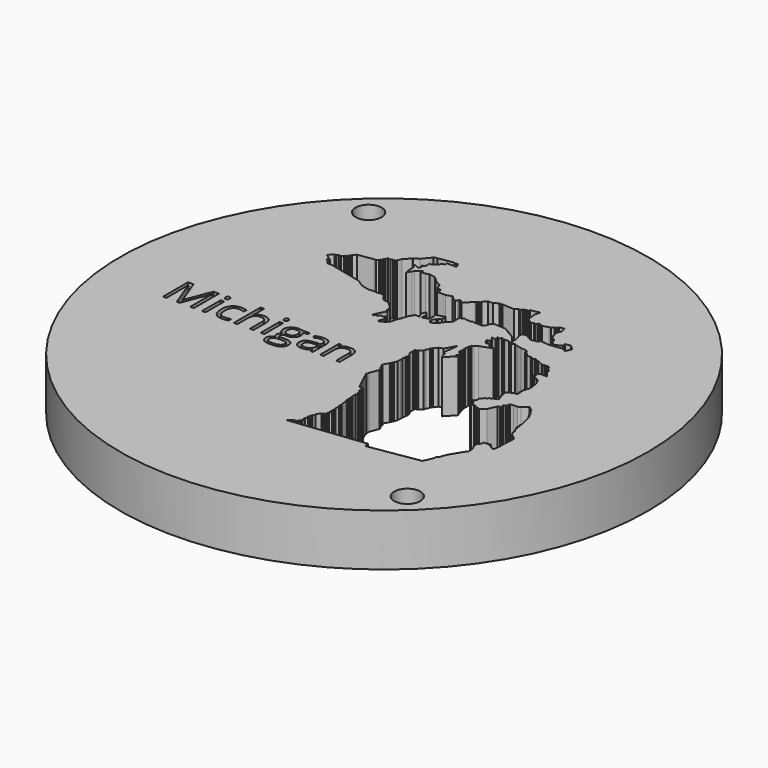
from build123d import *

# Parameters (mm, degrees)
F0_R         = 25.4
F0_R_2       = 1.25
F1_DEPTH     = 5
F2_TEXT_SIZE = 4.2111256337
F3_DEPTH     = 25


# Not quite as in the source:
# - Text() gives the source's letters only with a copy of the font that has no kerning and outlines rounded to 1/6400 em; it was checked with that copy


with BuildPart() as f1:
    # F0 (on Top) → F1 (new body)
    with BuildSketch(Plane.XY):
        Circle(F0_R)
        with Locations((15.783349916, -16.9354174861)):
            Circle(F0_R_2, mode=Mode.SUBTRACT)
        with Locations((-15.3492664, 17.3298159535)):
            Circle(F0_R_2, mode=Mode.SUBTRACT)
    extrude(amount=F1_DEPTH)

    # F2 (on face) → F3 (cut)
    with BuildSketch(Plane.XY.offset(5)):
        Polygon((-7.1277720854, 12.4056404456), (-7.3109893128, 12.8393787891), (-6.7987288348, 12.5963352621), (-6.6902944818, 12.9216387868), (-6.8395042811, 13.0705927815), (-6.5855989233, 13.1534645334), (-6.5736236811, 13.2494844339), (-6.5108160488, 13.3478995413), (-6.6192508675, 13.6918993667), (-6.3575119711, 13.6133776978), (-6.1593381688, 13.7953237279), (-5.796642974, 14.1817247495), (-5.5685560219, 14.3312895671), (-5.6059476919, 14.5182460546), (-5.0413394347, 14.5257245749), (-4.9815131351, 14.607985504), (-4.888035357, 14.5182460546), (-4.663687665, 14.5406806841), (-4.8581222072, 14.9893760681), (-4.9515999854, 14.7986812517), (-4.9927304499, 14.9519853294), (-5.0712525845, 14.8285934702), (-5.0824698992, 14.9220721796), (-5.2972559509, 14.9541556042), (-6.641685497, 14.735115692), (-6.7274633534, 14.6680477367), (-6.7821381753, 14.7193682406), (-6.9744680077, 14.6565940231), (-7.0342938416, 14.5444199443), (-7.6288152486, 13.826508075), (-8.0924667418, 13.5759860277), (-8.1448216866, 13.4778581533), (-8.6458576843, 12.9440743476), (-8.8066402823, 12.5514650717), (-8.9188143611, 12.4542480335), (-9.1095101088, 12.4617265537), (-9.2927273363, 12.3794656247), (-9.5656830817, 12.4093787745), (-9.6329879016, 12.2037269175), (-9.7414227203, 12.1027706191), (-9.7489003092, 11.9158150628), (-9.8573351279, 11.8709448725), (-9.8947267979, 11.7475539446), (-10.0913743195, 11.6190201435), (-10.2767857498, 11.6353798658), (-11.7455944419, 11.3960755989), (-12.0148109272, 11.1305983737), (-11.9587248191, 11.0072065145), (-12.0567845111, 11.0149033746), (-12.1308986992, 10.8987716958), (-12.0877359866, 10.7665282746), (-12.2728114948, 10.7828583568), (-12.3003042953, 10.6222052089), (-12.3801907504, 10.6257427085), (-12.5345503911, 10.4612940922), (-12.7769677552, 10.523354285), (-12.9007655011, 10.391465095), (-13.073738424, 10.3991246117), (-13.4813163299, 9.9649073364), (-13.1518466448, 9.7546427603), (-13.1106622391, 9.6284605448), (-12.9385474117, 9.6208390259), (-12.8557833095, 9.5680197237), (-13.0281141028, 9.384425357), (-13.0281141028, 9.3208597973), (-12.7850705758, 9.3283383176), (-12.7552073371, 9.1944148123), (-12.7252452075, 9.0105123818), (-12.628027238, 9.0591209009), (-12.5974396509, 8.9247867286), (-12.422375381, 8.9170346037), (-12.2466366738, 8.9394692332), (-9.0085528791, 8.1766871735), (-8.2644671202, 7.7018183656), (-7.505360331, 7.5182112386), (-7.1128155105, 7.5821662322), (-6.9782068022, 7.533557713), (-6.8809897639, 7.5859054923), (-6.7351637408, 7.4849487282), (-6.5631638281, 7.5933835469), (-5.8826426975, 7.4886879884), (-5.905077327, 7.2344271466), (-5.6844688952, 7.163383998), (-5.7442951947, 7.0512099192), (-5.6994254701, 6.9614709355), (-5.5909906514, 7.0175579749), (-5.5143811624, 6.8605176456), (-5.2619478665, 6.9016451016), (-5.127075726, 6.802898566), (-4.9927304499, 6.7969495431), (-4.2811993246, 6.0895033047), (-4.3982090428, 6.0379067436), (-4.3771734405, 5.9902025972), (-4.1589052416, 5.8808634058), (-4.3498775797, 5.7425163686), (-4.3245454219, 5.6649028218), (-4.1775836656, 5.658395121), (-4.6823825687, 4.6506910585), (-4.7160349786, 4.4824304059), (-4.6001221053, 4.4786911458), (-4.4909280854, 4.6080096089), (-4.3570785783, 4.6020825393), (-4.2486442253, 4.6510417404), (-4.1551659815, 4.8376475461), (-3.9420356043, 4.7441693023), (-3.7438618019, 4.8825168051), (-3.6466452293, 4.8899953254), (-3.5859393744, 4.7605300768), (-3.6802967079, 4.5721693896), (-3.6167316139, 4.4973869808), (-3.4922887951, 4.4772454448), (-3.7401227746, 4.2132129893), (-3.7401227746, 3.9963438176), (-3.6466452293, 3.9365179837), (-3.1156884506, 4.2917346582), (-3.0782972462, 4.4375606813), (-3.0118077362, 4.3613059405), (-2.9698626604, 4.4450387359), (-2.913775621, 4.6768649481), (-2.8142493157, 5.0720415796), (-2.6063358623, 5.4870885028), (-2.6290135387, 5.6262802047), (-2.5199085008, 5.7425163686), (-2.5199085008, 5.9331770969), (-2.4163748255, 6.0434777529), (-2.2987988717, 6.2781885764), (-2.206857817, 6.4617257707), (-2.0555970742, 6.4550277039), (-1.9404778719, 6.4926012709), (-1.8345903468, 6.4395580129), (-1.7658638535, 6.5127764829), (-1.9040555406, 6.7148180333), (-1.9479481664, 6.849297788), (-1.9479481664, 6.9602626832), (-1.9405520285, 7.1272877898), (-1.8653408393, 7.1239573185), (-1.8818918278, 7.1746668131), (-1.8032551743, 7.3316451162), (-1.6999338072, 7.1456425796), (-1.5803855445, 7.0857561167), (-1.5863857698, 6.9502545521), (-1.4583760701, 6.7865391851), (-1.5800438188, 6.7468282489), (-1.5573500666, 6.6772983409), (-1.5573500666, 6.481746644), (-1.482845441, 6.4784474604), (-0.980749129, 6.6423258494), (-0.9552610833, 7.2179159183), (-0.9789566164, 7.2905151173), (-1.0056832059, 7.4545583559), (-0.9320384706, 7.4512972496), (-0.7790197309, 7.4747815675), (-0.8082409775, 7.5643106398), (-0.7479685806, 7.5341178074), (-0.5664556183, 7.5260801241), (-0.5664556183, 7.589110377), (-0.4907736019, 7.5857590566), (-0.2429322236, 7.6666515962), (-0.1793213183, 7.6347863727), (-0.1543000981, 7.4812103994), (-0.2061939002, 7.226064815), (-0.3001260338, 7.1259932593), (-0.449858353, 7.041268316), (-0.43440721, 6.946431841), (-0.5207345239, 6.9502545521), (-0.7571360754, 6.5598915506), (-0.6467103836, 6.2215654728), (-0.2002567309, 6.3672827458), (0.1784821943, 6.7707761191), (0.1822209306, 6.867098103), (0.2464403923, 6.8642543629), (0.2464403923, 6.9636846874), (0.3542211489, 6.9988630712), (0.4108860674, 7.1022652657), (0.5433095946, 7.1454867628), (0.6159600453, 7.2905151173), (0.7133600134, 7.4849496596), (0.7133600134, 7.9710362479), (0.7133600134, 8.1713643005), (1.0088957017, 8.2678237074), (1.0683943983, 8.3711231127), (1.2371525816, 8.2739212758), (1.7028301691, 8.2533003299), (1.7958752097, 8.3524268121), (1.9324383323, 8.303240517), (2.6098789519, 8.2732423666), (2.8482188936, 8.2626882941), (2.9977834783, 8.4459055215), (3.1063242559, 8.6665134877), (3.1063242559, 8.8745476714), (3.2445664983, 8.8684260845), (3.3268267289, 9.0271973499), (4.5539315517, 8.9728591924), (4.6691740863, 8.8646868244), (4.9065817423, 8.7500038704), (5.0393473357, 8.6253834888), (5.1851733588, 8.5879918188), (5.7385643013, 8.225296624), (6.1982420617, 7.6441760164), (6.2475511422, 7.6419925317), (6.2475511422, 7.7891128468), (6.1702899561, 8.2633288028), (6.0969153571, 8.4881364532), (6.0338136705, 8.6814695969), (6.0338136705, 8.9506870136), (6.1021113827, 9.0800669876), (6.2957001332, 9.1116072516), (6.467693951, 9.1039910913), (6.588708179, 9.0680514739), (6.7256935872, 8.9394701645), (7.1332585067, 8.7300781161), (7.6636647912, 8.8476542689), (7.8586488962, 9.0553825721), (8.5541270673, 8.9581655338), (9.4111056205, 9.0477482697), (9.7643368556, 9.1052981345), (10.0198529102, 9.0939834764), (10.1897411068, 8.9345179752), (10.2965598926, 8.9693823829), (10.5206775908, 9.4694468884), (10.0705454504, 9.8919632773), (9.5451961372, 9.8063712374), (9.5837232329, 9.5698985083), (9.4552561641, 9.4330348074), (9.0289963409, 9.2012090608), (8.8638586256, 9.2994744612), (8.7186479941, 9.3059046194), (8.471865207, 9.8892077804), (8.1534511834, 10.0559782914), (8.1027867628, 10.2112057067), (8.021858283, 10.2871691982), (7.9875486617, 10.4977557899), (7.945951134, 10.7530743058), (7.9222135246, 10.8987716958), (8.0792568624, 11.272684671), (7.9633444548, 11.7475539446), (7.5043428103, 11.6727715358), (7.5043428103, 11.4633734855), (7.4228234148, 11.53989164), (7.3685416414, 11.4820619996), (7.4136923067, 11.3437278196), (7.3327413829, 11.377553428), (7.2731730027, 11.4334672689), (7.0700446908, 11.217062452), (6.9061564001, 11.2243196867), (6.3555194065, 11.0445981845), (6.0338136705, 11.1983342806), (5.9092761002, 11.157686668), (5.8133462444, 10.9473802149), (5.6002158672, 11.0445981845), (5.3963813696, 10.8987716958), (5.3646508604, 10.9959887341), (5.255064221, 11.037282278), (5.0898509598, 11.0445981845), (5.0617814995, 11.1305983737), (4.9234339967, 11.2315537408), (4.8241969579, 11.272684671), (4.8313166676, 11.4334672689), (4.8313166676, 11.7741720209), (4.7850860283, 11.9158150628), (4.7850860283, 12.1139883995), (4.9084774218, 12.6486830413), (4.0547203979, 12.4814710474), (4.0447395295, 12.2560756281), (3.89250259, 12.3719880357), (3.7772050798, 12.3343562711), (3.7717956785, 12.2121971321), (3.6879061236, 12.2909400358), (3.5810873378, 12.2560756281), (3.5309922063, 12.0151878316), (3.4640772008, 12.0779975801), (3.3268267289, 12.0840752497), (2.9977834783, 11.8647165536), (1.843838809, 11.9158150628), (1.7958752097, 11.8647165536), (1.7414368922, 11.9158150628), (1.5918718418, 11.9158150628), (1.1581330327, 11.6353798658), (0.7133600134, 11.6353798658), (0.3729162854, 11.272684671), (0.3430032812, 11.1305983737), (0.1822209306, 11.1305983737), (0.1522131088, 11.0299325805), (0.0697822926, 11.0030281221), (0, 10.9286848456), (-0.7338652504, 10.2107729763), (-0.8310825215, 10.2631207556), (-0.9544737404, 10.4500772431), (-1.1002997635, 10.4500772431), (-1.1703724623, 10.3105886297), (-1.3096907642, 10.1621644571), (-1.5517614229, 10.2978093725), (-1.8892555963, 10.6145981699), (-2.427689964, 10.4388594627), (-3.2615151722, 10.4388594627), (-3.2615151722, 10.5809466913), (-3.2199687064, 10.824676877), (-3.2989063766, 10.8987716958), (-3.467167262, 10.8576416969), (-3.5681235604, 10.8576416969), (-3.6466452293, 10.9698157758), (-3.6466452293, 11.0445981845), (-3.7940654162, 11.4105564617), (-3.882210236, 11.4932935685), (-4.2486442253, 11.6353798658), (-4.8581222072, 12.2074661776), (-5.4788170382, 12.334597297), (-5.777947139, 12.2224232182), (-6.2116859481, 12.1738146991), (-6.2415990978, 12.2747709975), (-6.1593381688, 12.3719880357), (-6.1855120584, 12.4392928556), (-6.2415990978, 12.4392928556), (-6.6753379069, 12.0130321011), (-6.8136854097, 11.8597280234), (-7.0342938416, 11.4334672689), (-7.1277720854, 11.8410317227), align=None)
        Polygon((6.0338136705, 7.542393636), (5.6002158672, 7.542393636), (5.6069437414, 7.5430339202), (5.5217761546, 7.5505487621), (5.3965300322, 7.4553615414), (5.2813035436, 7.6181814075), (5.2186804824, 7.6332110912), (5.1310081035, 7.322600577), (4.9606733955, 7.5280042365), (4.9105747603, 7.5229941867), (4.9005551264, 7.4628763832), (5.0157816149, 7.2875316255), (5.0182868727, 7.2098788805), (4.9882275052, 7.1823252365), (4.6225087717, 7.2148889303), (4.6149939299, 7.1597807109), (4.7202007845, 7.0846332237), (4.8203975894, 6.9593871012), (4.8404368572, 6.8792295642), (4.8203975894, 6.7915571854), (4.7252103686, 6.7038848065), (4.5724101365, 6.6412617452), (4.5849350281, 6.5535893664), (4.7402400523, 6.5385596827), (4.6049742959, 6.4483825117), (4.6475580893, 6.4108087681), (4.7649391927, 6.426311098), (4.7755665146, 6.1995913275), (4.9420637079, 6.2598134391), (5.1369010471, 6.2491861172), (5.3104832768, 6.0082962736), (5.4309284315, 6.0649760999), (5.5549158715, 6.0720611364), (5.8028902858, 5.9126489796), (4.6976315789, 5.4981769063), (4.4028456323, 5.3243418224), (4.2368546128, 5.2049090154), (4.2348303832, 5.1057189703), (4.1579073295, 4.9802134745), (4.178150557, 4.7595663927), (4.1153975762, 4.5713083819), (4.1821990162, 4.4680698775), (4.1356403381, 4.3951957487), (4.2379312217, 4.1565233842), (4.1491850279, 4.1450723074), (4.1491850279, 4.0735029615), (4.2894608341, 3.9761690423), (4.1033807211, 3.9275018498), (4.120557569, 3.8330305833), (4.2865979485, 3.7500101607), (4.3984507211, 3.6412249319), (4.3984507211, 3.4590300638), (4.3068421073, 3.3265247475), (4.3166573159, 3.2512748148), (4.4049941935, 3.2627258915), (4.5207337074, 3.2818648043), (4.5011597686, 3.2329298556), (3.693592269, 2.3596077226), (3.5124807619, 2.6782050263), (3.4941155463, 2.9522136319), (3.3290442079, 3.0575448181), (3.3290442079, 3.1188570429), (3.2881693915, 3.1565877143), (3.4521382768, 4.4436333701), (3.4232353792, 4.4658663683), (3.3832159825, 4.4347401708), (2.8985370882, 3.5498677753), (2.5072367862, 3.4231399186), (2.2448874079, 3.0740820803), (2.1759653464, 3.0629655812), (2.1826352458, 2.920674393), (2.0937032532, 2.9251209926), (2.0648003556, 2.8984413948), (2.0914799534, 2.8517520986), (2.1092663519, 2.7983931359), (1.9691984635, 2.6027427521), (1.9247325836, 2.3559564725), (1.6557134222, 2.1914325189), (1.5601116465, 2.1247335244), (1.5556650469, 2.0558112301), (1.4089273755, 2.0291316323), (1.3577914797, 1.9513162551), (1.3088790001, 1.8823940773), (1.3866943773, 1.7712290864), (1.342228381, 1.3532490702), (1.5023058513, 1.1865017004), (1.5934611438, 0.850783661), (1.5512183309, 0.8663467597), (1.5378786484, 0.8196574636), (1.5845679445, 0.7596284267), (1.5111990506, 0.7574051269), (1.4934126521, 0.6995993899), (1.5690047294, 0.6351236952), (1.5512184473, 0.5617548595), (1.4511699555, 0.4239103582), (1.5134223504, 0.321638654), (1.5089757508, 0.1126486022), (1.482296153, -0.0941181133), (1.4867427526, -0.254195591), (1.3690509368, -0.5000843666), (1.4099257533, -0.5692571867), (1.3784836046, -0.5692571867), (1.2967338553, -0.6384300068), (1.2967338553, -0.7610545726), (1.2244168902, -0.8145062602), (1.1866862187, -0.902544416), (0.9225718677, -1.3804655755), (0.9257160709, -1.4936574735), (1.0074657621, -1.5659744386), (1.1049364693, -1.5785513679), (1.0923596565, -1.720041153), (1.1080807308, -1.8049350474), (1.1741092894, -1.9212710904), (1.2788069434, -2.0220598672), (1.3087199768, -2.1865814924), (0.98341587, -3.042841563), (0.9310681489, -3.2522326801), (0.9310681489, -3.3756238408), (1.0544593679, -3.4391889349), (1.0357636493, -3.5588410683), (1.0619375389, -3.667275887), (1.3386328937, -4.243101459), (1.8695889739, -5.3199697286), (2.0303714555, -5.2077961154), (2.0116758533, -5.4209264927), (2.1575016435, -5.2601438947), (2.1088931244, -5.5331001058), (2.2696754895, -5.4433611222), (2.2061103955, -5.6415349245), (2.3369798437, -5.6340564042), (2.2173277102, -5.7798824273), (2.4379361421, -5.7574477978), (2.3033276666, -5.888317246), (2.3182842415, -5.9743169695), (2.4865448941, -6.0827517882), (2.3369798437, -6.1238822527), (2.4902839214, -6.2323166057), (2.404283965, -6.2884036452), (2.4715883192, -6.3557079993), (2.3743710481, -6.3930992037), (2.3855883628, -6.8530132994), (2.4753275793, -6.9165783934), (2.4005449377, -6.9726649672), (2.4005449377, -7.0736217313), (2.5201970711, -7.1110129356), (2.4155015126, -7.1409260854), (2.4117622524, -7.2231865488), (2.4940231815, -7.3054474778), (2.4304578546, -7.3428386822), (2.4192405399, -7.5036212802), (2.5052404962, -7.6905777678), (2.565066563, -8.2215331495), (2.6211533695, -8.3710988984), (2.5575882755, -8.4570981562), (2.580022905, -8.6440546438), (2.6660230942, -8.6702285334), (2.5688055903, -8.7786633521), (2.7071533259, -8.8310111314), (2.5912404526, -9.0590976179), (2.6585445739, -9.2161409557), (2.6361097116, -9.5339668915), (2.8193269391, -9.5863146707), (2.6323706843, -9.7171841189), (2.8492400888, -9.8106618971), (2.6323706843, -9.9078789353), (2.7968923096, -10.0985746831), (2.5725446176, -10.0985746831), (2.6248926297, -10.3191835806), (2.4753273465, -10.2705741301), (2.4790663738, -10.4164006189), (2.2995884065, -10.4089220986), (2.0415887702, -10.8426613733), (2.1612406708, -10.9697915614), (1.9518496701, -11.0632693395), (2.0715016872, -11.2165734172), (1.8658495974, -11.1754434183), (1.9368930953, -11.3698774949), (1.8209801055, -11.4932693541), (1.843838809, -11.5996661828), (1.9742839504, -11.6054425016), (1.8247189, -11.8185728788), (1.8209797563, -11.9643993676), (2.0266317297, -12.1214427054), (1.8247189, -12.1775288135), (1.8621101044, -12.2971814126), (1.7723711208, -12.2784860432), (1.6907415084, -12.3904054819), (1.6751538496, -12.5813549384), (1.5555018326, -12.5327464193), (1.3470466308, -12.5772578473), (0.9571245755, -12.915189378), (8.1167351454, -12.0969042182), (8.20020912, -12.5255505601), (13.0659369752, -11.7328064516), (13.3650666103, -11.0747199506), (13.4809799492, -10.8129810542), (13.4809799492, -10.5624590069), (13.6641971767, -10.4502858594), (13.6529793963, -10.39419882), (13.7240225449, -10.3530678898), (13.716544956, -10.2371554822), (13.9072397724, -9.7772423178), (14.4167490436, -8.9141351607), (14.6438479424, -8.5582872853), (14.8121090606, -8.3227222785), (14.7821949795, -7.8815054148), (14.6775003523, -7.5711579993), (14.5391523838, -7.4328100309), (14.5877609029, -7.354288362), (14.5437946463, -7.2417284788), (14.5840225741, -7.1411584504), (14.4426460471, -7.0388790589), (14.5989786834, -6.987853907), (14.7036742419, -6.8831583485), (14.7859351709, -6.7448108457), (14.79715202, -6.4942892641), (14.8569783196, -6.5354197286), (14.9990655482, -6.5167238936), (15.0813264772, -6.4643761143), (15.0962825865, -6.3970717601), (15.1972388849, -6.5279412083), (15.2794998139, -6.5428977832), (15.451499261, -6.4382022247), (15.5113255605, -6.6737672314), (15.6384557486, -6.6849845462), (15.6534127891, -6.7635066807), (15.8478468657, -6.797158625), (15.8702824265, -6.8943761289), (16.0235855728, -6.8756802939), (16.1072213047, -6.7234041787), (16.1500379582, -6.1988984235), (16.1500379582, -5.792296931), (16.2030644715, -4.5948126353), (16.0086303949, -4.460203927), (15.8254131675, -4.2844652198), (15.6608913094, -4.2470740154), (15.5861089006, -4.0414216928), (15.4851526022, -3.8918566424), (15.4963703826, -3.6076828837), (15.3804570436, -3.5067265853), (15.4103701934, -3.420726629), (15.2944568545, -3.3384659328), (15.3393270448, -3.2786396332), (15.2682829648, -3.2150745392), (15.2981961146, -3.1215965282), (15.1224574074, -2.99072708), (15.2234137058, -2.9196836986), (15.2383698151, -2.8262054548), (15.2388783099, -2.7274691521), (15.1448920369, -2.6392489672), (15.1935005561, -2.4597709998), (15.0626311079, -1.8577715382), (14.8495007306, -1.0725548491), (14.7261098027, -1.0575983906), (14.7298490629, -0.8332507568), (14.5989796147, -0.8220333839), (14.617674984, -0.6089031813), (14.3484584987, -0.4256859247), (14.4120231271, -0.3808164038), (14.400806278, -0.2649034723), (13.8698594999, 0.1708371509), (13.3800236508, -0.2536860993), (13.1444586441, -0.3733381454), (12.7723192073, -0.3879629357), (12.4489814043, -0.4406424414), (12.4067555633, -0.5870658893), (12.6284593716, -0.7285552565), (12.4452421442, -0.713598798), (12.2844595462, -0.7771638921), (12.1760247275, -0.9304681444), (12.2059378773, -1.2221201323), (12.0975030586, -1.1959462427), (11.9441989809, -1.28942437), (11.5815037861, -2.1008148324), (11.1402869225, -2.5009014644), (11.0206343234, -2.4223797955), (10.8598517254, -2.3550756741), (10.7028083876, -2.3812493309), (10.6616783887, -2.3214232642), (10.5495043099, -2.2204669658), (10.4186348617, -2.2092494182), (10.2578522637, -2.3700320162), (10.2615915239, -2.1980321035), (10.2354176342, -2.0970755722), (10.1269828156, -2.0522060804), (9.9549833685, -2.0933365449), (10.0484611467, -1.9923802465), (10.1008089259, -1.9138584612), (10.0559396669, -1.7904673005), (9.8278531805, -1.6371631064), (9.9662011489, -1.5848153271), (10.1045481861, -1.4277719893), (10.0596789271, -1.1548156617), (10.1120267063, -1.1473374907), (10.1232444867, -1.0351636447), (10.2690700442, -0.9790767217), (10.3475917131, -0.8182942402), (10.5008957908, -0.7734247483), (10.6387614303, -0.58988246), (10.8149824664, -0.5976858083), (10.8972433954, -0.4518597852), (11.0168950632, -0.4742945894), (11.2344093411, -0.3586394844), (11.2823732197, -0.238729539), (11.2188085914, -0.1489904971), (11.207590811, -0.0555123479), (11.1664608121, 0.0005745259), (11.1552430317, 0.1052701336), (11.0879391432, 0.165096164), (11.0767213628, 0.363269879), (11.0056782141, 0.4455306916), (11.0580259934, 0.5427479628), (11.001938954, 0.6549218087), (11.001938954, 0.8343999507), (11.2262871116, 1.0288344929), (11.6151561961, 1.1970952619), (11.8619380519, 1.2008344056), (11.8619380519, 1.4027472353), (11.7609817535, 1.4775297605), (11.8507212028, 1.5485732583), (11.8320249021, 1.6457905294), (11.7310686037, 1.7056165962), (11.820808053, 1.7654425465), (11.8320249021, 1.9037902821), (11.7609817535, 2.0047468133), (11.9292428717, 2.1281379741), (11.8694165722, 2.2889203392), (11.9795024442, 2.3936158977), (11.9795024442, 2.8844038445), (11.8955904618, 3.3994412515), (11.6741889079, 3.9046006776), (11.5590691566, 4.0126577951), (11.4086741042, 4.0782887363), (11.2075917423, 4.0126577951), (11.157387156, 4.0695373408), (11.2225478515, 4.1996142827), (10.94015781, 4.2787180601), (10.9159396961, 4.3529183604), (11.072983034, 4.5735272579), (10.8448965475, 4.603439942), (10.949592106, 4.6632662416), (10.9533304349, 4.8240483738), (11.1028961837, 4.7230920754), (11.1337667294, 4.8606255771), (11.7908949032, 4.8315268941), (11.6076786071, 5.0633526407), (11.5029830486, 5.2316132933), (11.3795911893, 5.3587434813), (11.3384611905, 5.4896129295), (11.3683743402, 5.6242216378), (11.3309826702, 5.7139606215), (11.1814178526, 5.7513518259), (11.0655045137, 5.8523081243), (11.0056791455, 6.1177862808), (10.8448965475, 6.0654385015), (10.7925487682, 6.2150037847), (10.6392446905, 6.0729170218), (10.4859406129, 6.2150037847), (10.4298535734, 6.0841343366), (10.3438533843, 6.20378647), (10.3198008538, 6.0920807669), (9.7139459813, 6.3955774843), (9.5960283652, 6.3570905477), (9.4726374373, 6.5029165708), (9.3006370589, 6.536568515), (9.1361161321, 6.4056990668), (9.094985202, 6.5141338855), (8.8781164959, 6.5814382397), (8.7734209374, 6.5477858298), (8.4626258097, 6.5400058326), (8.4368987009, 6.6188294441), (8.2648992538, 6.8768290803), (8.0298499518, 6.8930749971), (8.1041166559, 7.0787421428), (7.9633444548, 7.1862910422), (7.3600304313, 7.2395242751), (6.9300308824, 7.3516983539), (6.5935095772, 7.4863065965), (6.361683365, 7.2905151173), (6.2981182709, 7.5461328961), (6.0755655613, 7.4144727398), align=None)
        with Locations((-19.2612486653, -3.0320104563)):
            Text('Michigan', F2_TEXT_SIZE, font='Open Sans', text_align=(TextAlign.LEFT, TextAlign.BOTTOM))
    extrude(amount=-F3_DEPTH, mode=Mode.SUBTRACT)


solid = f1.part
